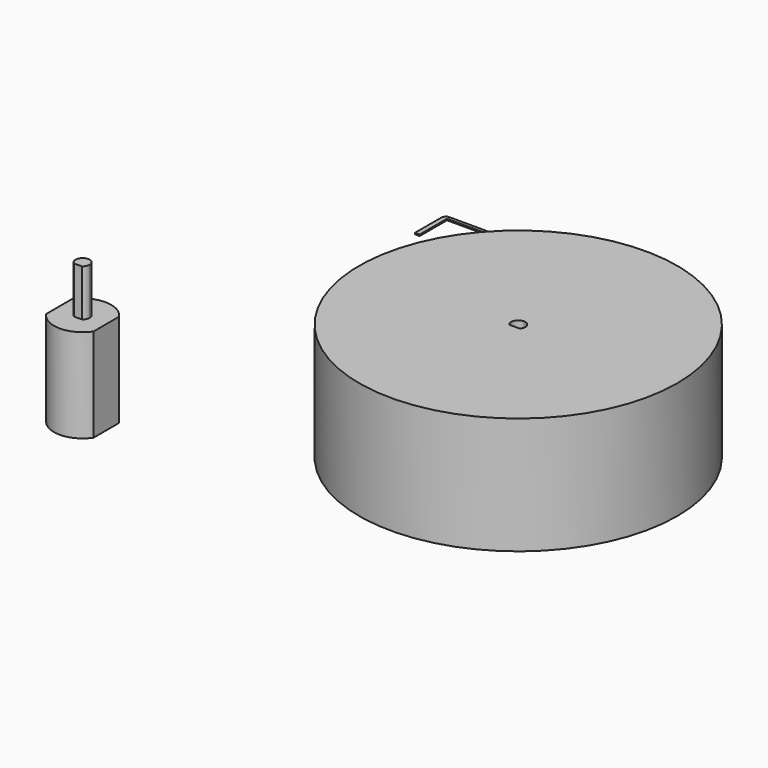
from build123d import *

# Parameters (mm, degrees)
F0_R     = 34
F1_DEPTH = 25
F2_W     = 10.1202055069
F2_H     = 6.8258544885
F3_DEPTH = 20
F5_DEPTH = 10
F6_W     = 10
F6_H     = 0.7
F7_DEPTH = 0.3
F9_DEPTH = 8


with BuildPart() as f1:
    # F0 (on Top) → F1 (new body)
    with BuildSketch(Plane.XY):
        Circle(F0_R)
        with BuildLine():
            ThreePointArc((0, 1.5), (1.0606601718, 1.0606601718), (1.5, 0))
            ThreePointArc((1.5, 0), (1.4012585384, -0.5352331347), (1.1180339887, -1))
            ThreePointArc((1.1180339887, -1), (0, -1.5), (-1.1180339887, -1))
            ThreePointArc((-1.1180339887, -1), (-1.3693063938, 0.6123724357), (0, 1.5))
        make_face(mode=Mode.SUBTRACT)
        with BuildLine():
            ThreePointArc((-1.1180339887, -1), (0, -1.5), (1.1180339887, -1))
            Line((1.1180339887, -1), (0, -1))
            Line((0, -1), (-1.1180339887, -1))
        make_face()
    extrude(amount=F1_DEPTH)

    # F8 (on face) → F9 (cut)
    with BuildSketch(Plane.XZ.offset(-52.1748177707)):
        with BuildLine():
            ThreePointArc((-63.1654030268, 0.15), (-63.2093370096, 0.2560660172), (-63.3154030268, 0.3))
            Line((-63.3154030268, 0.3), (-63.3154030268, 0))
            ThreePointArc((-63.3154030268, 0), (-63.2093370096, 0.0439339828), (-63.1654030268, 0.15))
        make_face()
        with BuildLine():
            Line((-63.3154030268, 0), (-63.3154030268, 0.3))
            ThreePointArc((-63.3154030268, 0.3), (-63.4654030268, 0.15), (-63.3154030268, 0))
        make_face()
    extrude(amount=F9_DEPTH, mode=Mode.SUBTRACT)


with BuildPart() as f3:
    # F2 (on Top) → F3 (new body)
    with BuildSketch(Plane.XY):
        with BuildLine():
            Line((-69.9120647834, -31.9230046827), (-59.7918592765, -31.9230046827))
            ThreePointArc((-59.7918592765, -31.9230046827), (-64.8519620299, -29.232431927), (-69.9120647834, -31.9230046827))
        make_face()
        with Locations((-64.8519620299, -35.335931927)):
            Rectangle(F2_W, F2_H)
        with BuildLine():
            ThreePointArc((-69.9120647834, -38.7488591712), (-64.8519620299, -41.439431927), (-59.7918592765, -38.7488591712))
            Line((-59.7918592765, -38.7488591712), (-69.9120647834, -38.7488591712))
        make_face()
    extrude(amount=F3_DEPTH)

    # F4 (on face) → F5 (join)
    with BuildSketch(Plane.XY.offset(20)):
        with BuildLine():
            ThreePointArc((-64.0228058323, -36.585931927), (-63.5302710115, -36.0452505097), (-63.3519620299, -35.335931927))
            ThreePointArc((-63.3519620299, -35.335931927), (-65.5612806127, -34.0142409085), (-65.6811182275, -36.585931927))
            Line((-65.6811182275, -36.585931927), (-65.605327487, -36.585931927))
            Line((-65.605327487, -36.585931927), (-64.8519620299, -36.585931927))
            Line((-64.8519620299, -36.585931927), (-64.0228058323, -36.585931927))
        make_face()
    extrude(amount=F5_DEPTH)


with BuildPart() as f7:
    # F6 (on Top) → F7 (new body)
    with BuildSketch(Plane.XY):
        with BuildLine():
            Line((-62.8154030268, 59.4748177707), (-62.8154030268, 60.1748177707))
            ThreePointArc((-62.8154030268, 60.1748177707), (-63.5225098079, 59.8819245519), (-63.8154030268, 59.1748177707))
            Line((-63.8154030268, 59.1748177707), (-63.8154030268, 52.1748177707))
            Line((-63.8154030268, 52.1748177707), (-62.8154030268, 52.1748177707))
            Line((-62.8154030268, 52.1748177707), (-62.8154030268, 59.4748177707))
        make_face()
        with BuildLine():
            ThreePointArc((-51.8154030268, 59.1748177707), (-52.1082962456, 59.8819245519), (-52.8154030268, 60.1748177707))
            Line((-52.8154030268, 60.1748177707), (-52.8154030268, 59.4748177707))
            Line((-52.8154030268, 59.4748177707), (-52.8154030268, 52.1748177707))
            Line((-52.8154030268, 52.1748177707), (-51.8154030268, 52.1748177707))
            Line((-51.8154030268, 52.1748177707), (-51.8154030268, 59.1748177707))
        make_face()
        with Locations((-57.8154030268, 59.8248177707)):
            Rectangle(F6_W, F6_H)
    extrude(amount=F7_DEPTH)


solid = Compound([f1.part, f3.part, f7.part])
